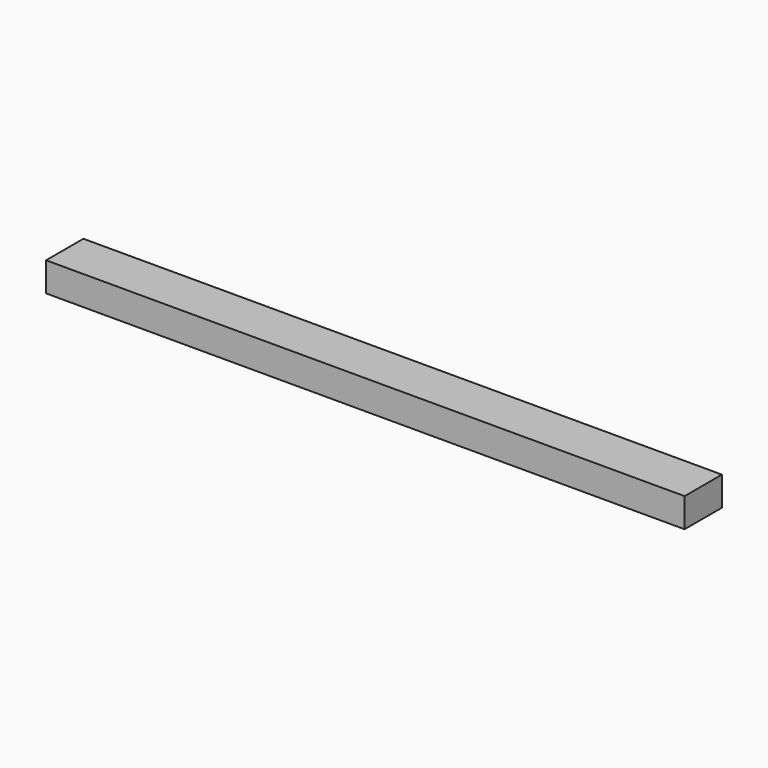
from build123d import *

# Parameters (mm, degrees)
F0_W     = 406.4
F0_H     = 254
F1_DEPTH = 5562.6


with BuildPart() as f1:
    # F0 (on Right) → F1 (new body)
    with BuildSketch(Plane.YZ):
        Rectangle(F0_W, F0_H)
    extrude(amount=F1_DEPTH)


solid = f1.part
